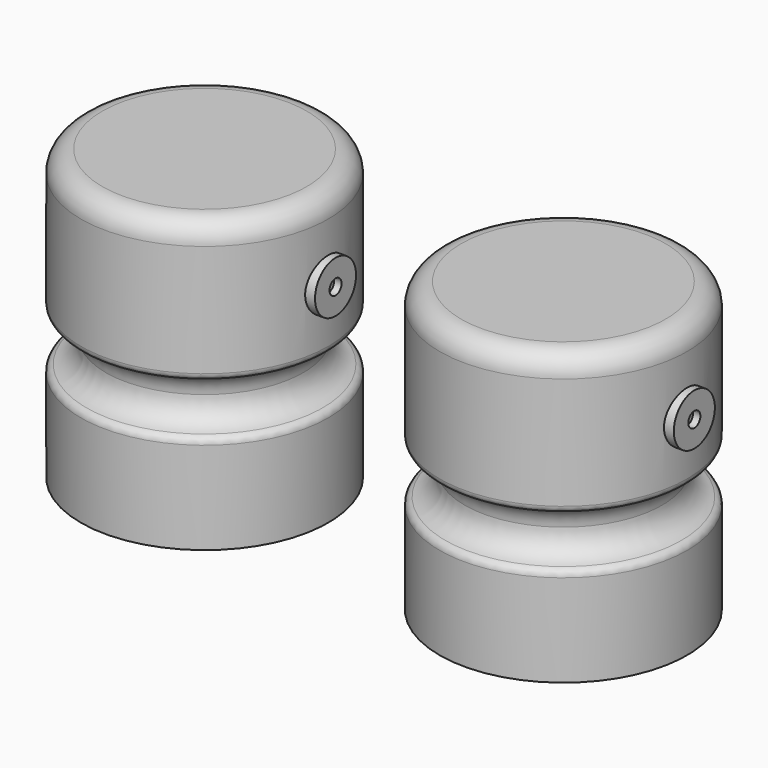
from build123d import *

# Parameters (mm, degrees)
F0_W     = 31.5
F0_H     = 1.5
F2_R     = 6
F4_R     = 2
F5_R     = 7.15
F5_R_2   = 2.1
F6_DEPTH = 36.5


# Not quite as in the source:
# - a fillet or chamfer that OpenCascade refuses, or shapes differently, is made with other operations: its cross-section is extruded or revolved along the edge and cut away or added


with BuildPart() as f1:
    # F0 (on Front) → F1 (revolve)
    with BuildSketch(Plane.XZ):
        with Locations((-15.75, -0.75)):
            Rectangle(F0_W, F0_H)
        Polygon((-31.5, 0), (0, 0), (0, 80.5), (-34.5, 80.5), (-34.5, 41.5), (-27.5, 41.5), (-27.5, 27.5), (-34.5, 27.5), (-34.5, 0), align=None)
    revolve(axis=Axis((0, 0, 39.7997796935), (0, 0, 1)))

    # F2
    f2_edges = [f1.edges().sort_by_distance(p)[0] for p in [
        (34.5, 0, 80.5),
    ]]
    fillet(f2_edges, radius=F2_R)

    # F3: fillet of radius 7 on 2 edges, made by hand

    # F3_s1 → F3_t2 (revolve)
    with BuildSketch(Plane.XZ):
        with BuildLine():
            ThreePointArc((-27.5, 34.5), (-29.5502525317, 29.5502525317), (-34.5, 27.5))
            Line((-34.5, 27.5), (-27.5, 27.5))
            Line((-27.5, 27.5), (-27.5, 34.5))
        make_face()
    revolve(axis=Axis((0, 0, 27.5), (0, 0, 1)))

    # F3_s3 → F3_t4 (revolve)
    with BuildSketch(Plane.XZ):
        with BuildLine():
            ThreePointArc((-34.5, 41.5), (-29.5502525317, 39.4497474683), (-27.5, 34.5))
            Line((-27.5, 34.5), (-27.5, 41.5))
            Line((-27.5, 41.5), (-34.5, 41.5))
        make_face()
    revolve(axis=Axis((0, 0, 41.5), (0, 0, 1)))

    # F4
    f4_edges = [f1.edges().sort_by_distance(p)[0] for p in [
        (34.5, 0, 41.5),
        (34.5, 0, 27.5),
    ]]
    fillet(f4_edges, radius=F4_R)

    # F5 (on Right) → F6 (join)
    with BuildSketch(Plane.YZ):
        with Locations((0, 58.5)):
            Circle(F5_R)
        with Locations((0, 58.5)):
            Circle(F5_R_2, mode=Mode.SUBTRACT)
    extrude(amount=F6_DEPTH)


with BuildPart() as f7_1:
    # F7: copy of F1
    add(f1.part.moved(Location((100, 0, 0))))


solid = Compound([f1.part, f7_1.part])
